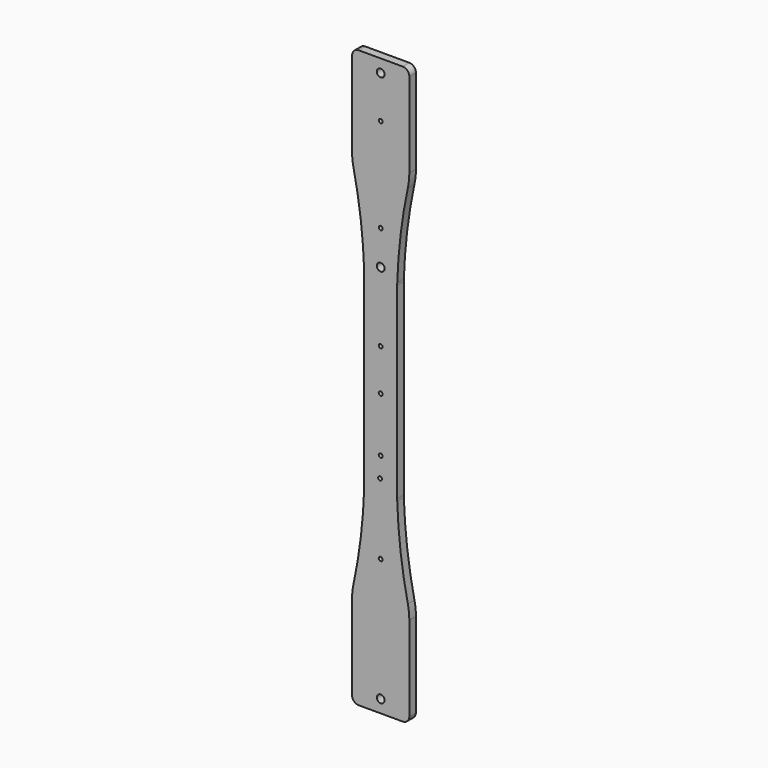
from build123d import *

# Parameters (mm, degrees)
F0_R        = 1.5
F0_R_2      = 3
F1_DEPTH    = 6.35
F2_R        = 5.08
F3_T1_DEPTH = 6.35
F3_T3_DEPTH = 34.0624500619


# Not quite as in the source:
# - a fillet or chamfer that OpenCascade refuses, or shapes differently, is made with other operations: its cross-section is extruded or revolved along the edge and cut away or added
# - a feature names something its author has since deleted; it is built from what else it names


with BuildPart() as f1:
    # F0 (on Front) → F1 (new body)
    with BuildSketch(Plane.XZ):
        Polygon((-12.7, 104.7939062119), (-12.7, -41.3571195934), (-12.7, -95.0903743505), (12.7, -95.0903743505), (12.7, -41.3571195934), (12.7, 104.7939062119), (12.7, 162.231490016), (0, 162.231490016), (-12.7, 162.231490016), align=None)
        with Locations((-0.4384766798, -31.0452261312)):
            Circle(F0_R, mode=Mode.SUBTRACT)
        with Locations((0, -85.4520261312)):
            Circle(F0_R, mode=Mode.SUBTRACT)
        with Locations((0, -15.4520261312)):
            Circle(F0_R, mode=Mode.SUBTRACT)
        with Locations((0, 26.5547856688)):
            Circle(F0_R, mode=Mode.SUBTRACT)
        with BuildLine():
            ThreePointArc((1.5, 58.5587856688), (-1.0606601718, 57.4981254971), (0, 60.0587856688))
            ThreePointArc((0, 60.0587856688), (1.0606601718, 59.6194458406), (1.5, 58.5587856688))
        make_face(mode=Mode.SUBTRACT)
        with BuildLine():
            ThreePointArc((0, 109.0876222849), (-3, 112.0876222849), (0, 115.0876222849))
            ThreePointArc((0, 115.0876222849), (2.1213203436, 114.2089426284), (3, 112.0876222849))
            ThreePointArc((3, 112.0876222849), (2.1213203436, 109.9663019413), (0, 109.0876222849))
        make_face(mode=Mode.SUBTRACT)
        with BuildLine():
            ThreePointArc((0, 137.0615974688), (-1.5, 138.5615974688), (0, 140.0615974688))
            ThreePointArc((0, 140.0615974688), (1.0606601718, 139.6222576406), (1.5, 138.5615974688))
            ThreePointArc((1.5, 138.5615974688), (1.0606601718, 137.5009372971), (0, 137.0615974688))
        make_face(mode=Mode.SUBTRACT)
        with BuildLine():
            ThreePointArc((-22, 177.5426715612), (-15.5787747464, 141.3947174009), (-12.7, 104.7939062119))
            Line((-12.7, 104.7939062119), (-12.7, 162.231490016))
            Line((-12.7, 162.231490016), (0, 162.231490016))
            Line((0, 162.231490016), (0, 177.1979365494))
            Line((0, 177.1979365494), (0, 209.4587856688))
            ThreePointArc((0, 209.4587856688), (-1.5, 210.9587856688), (0, 212.4587856688))
            Line((0, 212.4587856688), (0, 240.5199192026))
            ThreePointArc((0, 240.5199192026), (-3, 243.5199192026), (0, 246.5199192026))
            Line((0, 246.5199192026), (0, 253.3979365494))
            Line((0, 253.3979365494), (-4.6853246795, 253.3979365494))
            Line((-4.6853246795, 253.3979365494), (-22, 253.3979365494))
            Line((-22, 253.3979365494), (-22, 236.307715069))
            Line((-22, 236.307715069), (-22, 225.4278063774))
            Line((-22, 225.4278063774), (-22, 177.5426715612))
        make_face()
        with BuildLine():
            Line((12.7, 162.231490016), (12.7, 104.7939062119))
            ThreePointArc((12.7, 104.7939062119), (15.5787747464, 141.3947174009), (22, 177.5426715612))
            Line((22, 177.5426715612), (22, 225.4278063774))
            Line((22, 225.4278063774), (22, 236.307715069))
            Line((22, 236.307715069), (22, 253.3979365494))
            Line((22, 253.3979365494), (4.6853246795, 253.3979365494))
            Line((4.6853246795, 253.3979365494), (0, 253.3979365494))
            Line((0, 253.3979365494), (0, 246.5199192026))
            ThreePointArc((0, 246.5199192026), (2.1213203436, 245.6412395461), (3, 243.5199192026))
            ThreePointArc((3, 243.5199192026), (2.1213203436, 241.398598859), (0, 240.5199192026))
            Line((0, 240.5199192026), (0, 212.4587856688))
            ThreePointArc((0, 212.4587856688), (1.0606601718, 212.0194458406), (1.5, 210.9587856688))
            ThreePointArc((1.5, 210.9587856688), (1.0606601718, 209.8981254971), (0, 209.4587856688))
            Line((0, 209.4587856688), (0, 177.1979365494))
            Line((0, 177.1979365494), (0, 162.231490016))
            Line((0, 162.231490016), (12.7, 162.231490016))
        make_face()
        with BuildLine():
            Line((-22, -189.9611499309), (-4.6853246795, -189.9611499309))
            ThreePointArc((-4.6853246795, -189.9611499309), (-10.3525559476, -187.6137058785), (-12.7, -181.9464746103))
            Line((-12.7, -181.9464746103), (-12.7, -113.7611499309))
            Line((-12.7, -113.7611499309), (12.7, -113.7611499309))
            Line((12.7, -113.7611499309), (12.7, -181.9464746103))
            ThreePointArc((12.7, -181.9464746103), (10.3525559476, -187.6137058785), (4.6853246795, -189.9611499309))
            Line((4.6853246795, -189.9611499309), (22, -189.9611499309))
            Line((22, -189.9611499309), (22, -172.8709284505))
            Line((22, -172.8709284505), (22, -161.9910197589))
            Line((22, -161.9910197589), (22, -114.1058849427))
            ThreePointArc((22, -114.1058849427), (15.5787747464, -77.9579307824), (12.7, -41.3571195934))
            Line((12.7, -41.3571195934), (12.7, -95.0903743505))
            Line((12.7, -95.0903743505), (-12.7, -95.0903743505))
            Line((-12.7, -95.0903743505), (-12.7, -41.3571195934))
            ThreePointArc((-12.7, -41.3571195934), (-15.5787747464, -77.9579307824), (-22, -114.1058849427))
            Line((-22, -114.1058849427), (-22, -161.9910197589))
            Line((-22, -161.9910197589), (-22, -172.8709284505))
            Line((-22, -172.8709284505), (-22, -189.9611499309))
        make_face()
        with BuildLine():
            ThreePointArc((-12.7, -181.9464746103), (-10.3525559476, -187.6137058785), (-4.6853246795, -189.9611499309))
            Line((-4.6853246795, -189.9611499309), (0, -189.9611499309))
            Line((0, -189.9611499309), (4.6853246795, -189.9611499309))
            ThreePointArc((4.6853246795, -189.9611499309), (10.3525559476, -187.6137058785), (12.7, -181.9464746103))
            Line((12.7, -181.9464746103), (12.7, -113.7611499309))
            Line((12.7, -113.7611499309), (-12.7, -113.7611499309))
            Line((-12.7, -113.7611499309), (-12.7, -181.9464746103))
        make_face()
        with Locations((0, -180.0831407309)):
            Circle(F0_R_2, mode=Mode.SUBTRACT)
    extrude(amount=F1_DEPTH)

    # F2
    f2_edges = [f1.edges().sort_by_distance(p)[0] for p in [
        (-22, -3.175, 253.397937),
        (22, -3.175, 253.397937),
        (22, -3.175, -189.96115),
        (-22, -3.175, -189.96115),
    ]]
    fillet(f2_edges, radius=F2_R)

    # F3: fillet of radius 50.8 on 8 edges, made by hand

    # F3_s2 → F3_t1 (join)
    with BuildSketch(Plane.XZ):
        with BuildLine():
            ThreePointArc((-12.7261251288, 105.6376323271), (-12.7065317021, 104.8232386677), (-12.7, 104.0086355302))
            Line((-12.7, 104.0086355302), (-12.7, 104.7939062119))
            ThreePointArc((-12.7, 104.7939062119), (-12.7128266876, 105.2157765732), (-12.7261251288, 105.6376323271))
        make_face()
        with BuildLine():
            ThreePointArc((12.7261251288, 105.6376323271), (12.7065317021, 104.8232386677), (12.7, 104.0086355302))
            Line((12.7, 104.0086355302), (12.7, 104.7939062119))
            ThreePointArc((12.7, 104.7939062119), (12.7128266876, 105.2157765732), (12.7261251288, 105.6376323271))
        make_face()
        with BuildLine():
            ThreePointArc((12.7, -40.5718489117), (12.7065317021, -41.3864520492), (12.7261251288, -42.2008457086))
            ThreePointArc((12.7261251288, -42.2008457086), (12.7128266876, -41.7789899547), (12.7, -41.3571195934))
            Line((12.7, -41.3571195934), (12.7, -40.5718489117))
        make_face()
        with BuildLine():
            ThreePointArc((-12.7, -40.5718489116), (-12.7065317021, -41.3864520492), (-12.7261251288, -42.2008457086))
            ThreePointArc((-12.7261251288, -42.2008457086), (-12.7128266876, -41.7789899547), (-12.7, -41.3571195934))
            Line((-12.7, -41.3571195934), (-12.7, -40.5718489116))
        make_face()
    extrude(amount=F3_T1_DEPTH)

    # F3_s4 → F3_t3 (cut)
    with BuildSketch(Plane.XZ.offset(-13.856225031)):
        with BuildLine():
            ThreePointArc((-20.8768334444, -109.025182453), (-21.7184280188, -114.3071737314), (-22, -119.6483749551))
            Line((-22, -119.6483749551), (-22, -114.1058849427))
            ThreePointArc((-22, -114.1058849427), (-21.429661091, -111.5674692633), (-20.8768334444, -109.025182453))
        make_face()
        with BuildLine():
            ThreePointArc((20.8768334444, -109.025182453), (21.7184280188, -114.3071737314), (22, -119.6483749551))
            Line((22, -119.6483749551), (22, -114.1058849427))
            ThreePointArc((22, -114.1058849427), (21.429661091, -111.5674692633), (20.8768334444, -109.025182453))
        make_face()
        with BuildLine():
            ThreePointArc((22, 183.0851615736), (21.7184280188, 177.7439603499), (20.8768334444, 172.4619690715))
            ThreePointArc((20.8768334444, 172.4619690715), (21.429661091, 175.0042558818), (22, 177.5426715612))
            Line((22, 177.5426715612), (22, 183.0851615736))
        make_face()
        with BuildLine():
            ThreePointArc((-22, 183.0851615736), (-21.7184280188, 177.7439603499), (-20.8768334444, 172.4619690715))
            ThreePointArc((-20.8768334444, 172.4619690715), (-21.429661091, 175.0042558818), (-22, 177.5426715612))
            Line((-22, 177.5426715612), (-22, 183.0851615736))
        make_face()
    extrude(amount=F3_T3_DEPTH, mode=Mode.SUBTRACT)


solid = f1.part
